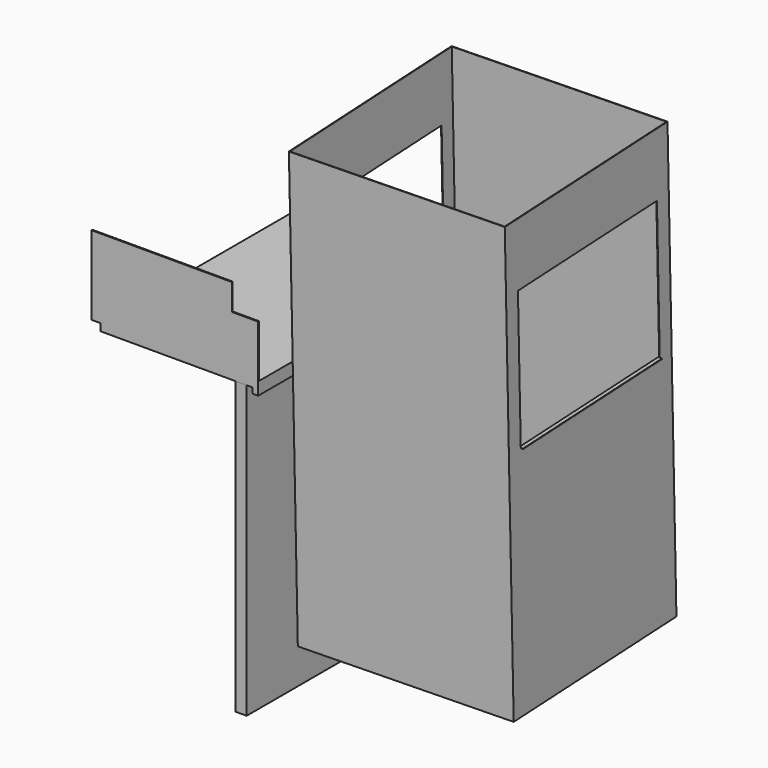
from build123d import *

# Parameters (mm, degrees)
F2_DEPTH  = 457.2
F3_W      = 441.325
F3_H      = 796.925
F4_DEPTH  = 15.875
F11_DEPTH = 3.175
F13_W     = 774.7
F13_H     = 842.9625
F14_DEPTH = 31.75
F17_DEPTH = 1.5875
F21_DEPTH = 1.5875
F23_W     = 392.1125
F23_H     = 842.9625
F24_DEPTH = 19.05
F25_W     = 50.8
F25_H     = 22.225
F26_DEPTH = 392.1125
F28_DEPTH = 1.524


with BuildPart() as f2:
    # F1 (on Right) → F2 (new body)
    with BuildSketch(Plane.YZ):
        with BuildLine():
            Line((393.7, 0), (-406.4, 0))
            Line((-406.4, 0), (-406.4, -36.5125))
            Line((-406.4, -36.5125), (406.4, -36.5125))
            Line((406.4, -36.5125), (406.4, -12.7))
            ThreePointArc((406.4, -12.7), (402.6802561211, -3.7197438789), (393.7, 0))
        make_face()
    extrude(amount=F2_DEPTH)

    # F3 (on face) → F4 (cut)
    with BuildSketch(Plane(origin=(0, 0, -36.5125), x_dir=(1, 0, 0), z_dir=(0, 0, -1))):
        with Locations((220.6625, 7.9375)):
            Rectangle(F3_W, F3_H)
    extrude(amount=-F4_DEPTH, mode=Mode.SUBTRACT)

    # F10 (on offset) → F11 (join)
    with BuildSketch(Plane.XZ.offset(406.4)):
        Polygon((274.5299355409, 0), (457.2, 0), (457.2, 152.4), (381, 152.4), (381, 228.6), (-25.4, 228.6), (-25.4, 0), align=None)
    extrude(amount=-F11_DEPTH)


with BuildPart() as f14:
    # F13 (on offset) → F14 (new body)
    with BuildSketch(Plane.YZ.offset(423.8625)):
        with Locations((-19.05, -442.11875)):
            Rectangle(F13_W, F13_H)
    extrude(amount=-F14_DEPTH)

    # F23 (on face) → F24 (join)
    with BuildSketch(Plane(origin=(0, 368.3, 0), x_dir=(-1, 0, 0), z_dir=(0, 1, 0))):
        with Locations((-196.05625, -442.11875)):
            Rectangle(F23_W, F23_H)
    extrude(amount=-F24_DEPTH)

    # F25 (on face) → F26 (join, through all)
    with BuildSketch(Plane(origin=(392.1125, 0, 0), x_dir=(0, -1, 0), z_dir=(-1, 0, 0))):
        with Locations((-323.85, -31.75)):
            Rectangle(F25_W, F25_H)
    extrude(amount=F26_DEPTH)


with BuildPart() as f17:
    # F16 (on offset) → F17 (new body)
    with BuildSketch(Plane(origin=(477.6201094775, 12.5069227266, 0), x_dir=(0.0261769483, -0.999657325, 0), z_dir=(-0.999657325, -0.0261769483, 0))):
        Polygon((-266.9286201536, 580.3113605768), (-300.3395681263, -695.6012661558), (309.0515371788, -711.5587338442), (342.4624851515, 564.3538928883), align=None)
        Polygon((282.5689202331, -24.8301750237), (-237.9526488816, -11.1998380398), (-227.3143370893, 395.0608988303), (293.2072320255, 381.4305618463), align=None, mode=Mode.SUBTRACT)
    extrude(amount=F17_DEPTH)


with BuildPart() as f18_1:
    # F18: instance of F17
    add(f17.part.mirror(Plane(origin=(782.32, 20.32, -101.6), x_dir=(0.0261769483, -0.999657325, 0), z_dir=(-0.999657325, -0.0261769483, 0))))


with BuildPart() as f17_1:
    add(f17.part)

    add(f18_1.part)  # F21 merges F18_1
    # F20 (on plane+point) → F21 (join)
    with BuildSketch(Plane(origin=(-7.3801007247, 281.8346761317, 7.3826305678), x_dir=(0.9996575598, 0.0261590049, 0.0006852325), z_dir=(0.0261679781, -0.9993147674, -0.0261769483))):
        Polygon((1086.9015409083, -703.9700752338), (1087.776437166, 572.3796249098), (478.176580381, 572.7974858089), (477.3016841234, -703.5522143346), align=None)
    extrude(amount=F21_DEPTH)


with BuildPart() as f22_1:
    # F22: instance of F17
    add(f17_1.part.mirror(Plane(origin=(782.8423262467, 0.3731653894, -101.6), x_dir=(0.0006852326, -0.0261679781, 0.999657325), z_dir=(0.0261679781, -0.9993147674, -0.0261769483))))


with BuildPart() as f17_2:
    add(f17_1.part)

    add(f22_1.part)  # F28 merges F22_1
    # F27 (on face) → F28 (join)
    with BuildSketch(Plane(origin=(-0.0119400923, 0.4559737301, -17.4189032553), x_dir=(0.9999997652, 1.79312e-05, -0.000684998), z_dir=(0.0006852326, -0.0261679781, 0.999657325))):
        Polygon((1091.2462910804, -254.6535570042), (1102.3549857122, -254.3627652791), (1088.7293163055, 266.1589260396), (1077.6206216737, 265.8681343144), align=None)
    extrude(amount=F28_DEPTH)

    # F29: F17 across plane


with BuildPart() as f17_3:
    add(f17_2.part)
    add(f17_2.part.mirror(Plane(origin=(782.32, 20.32, -101.6), x_dir=(0.0261769483, -0.999657325, 0), z_dir=(-0.999657325, -0.0261769483, 0))))


solid = Compound([f2.part, f14.part, f17_3.part])
